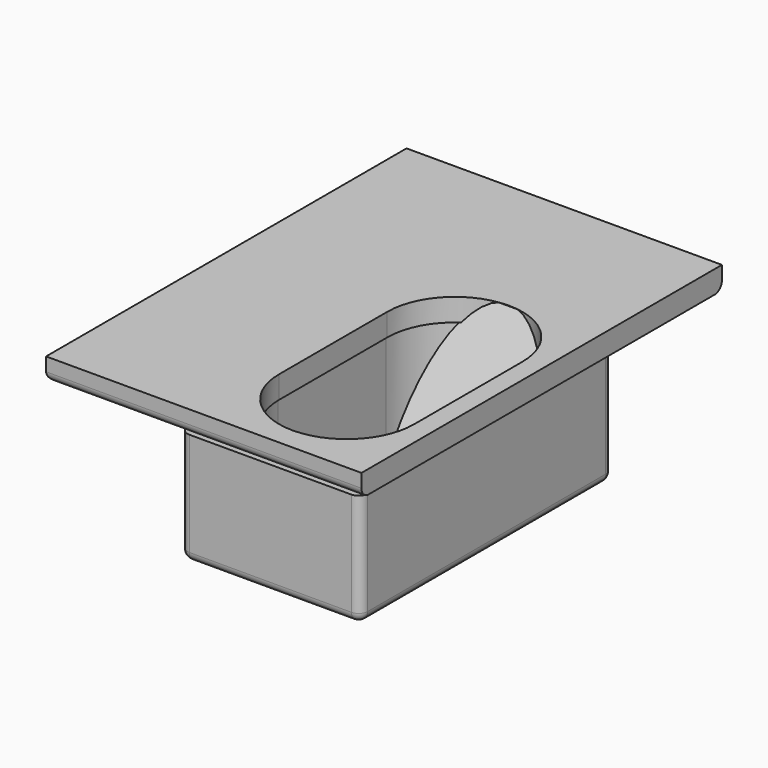
from build123d import *

# Parameters (mm, degrees)
F2_W     = 19.05
F2_H     = 25.4
F2_W_2   = 15.875
F2_H_2   = 19.05
F2_H_3   = 6.35
F2_W_3   = 6.35
F3_DEPTH = 3.175
F1_W     = 19.05
F1_H     = 6.35
F1_W_2   = 6.35
F1_H_2   = 19.05
F4_DEPTH = 15.875
F5_R     = 3.175
F6_DEPTH = 12.7
F9_DEPTH = 19.05
F10_R    = 1.27
F10_2_R  = 1.27


# Not quite as in the source:
# - a feature of the source that left no trace in its solid (it failed there, or was rolled back) is left out


with BuildPart() as f3:
    # F2 (on Top) → F3 (new body)
    with BuildSketch(Plane.XY):
        Polygon((0, 31.75), (-22.225, 31.75), (-22.225, 0), (-3.175, 0), (-3.175, 12.7), (0, 12.7), align=None)
        with Locations((-12.7, -19.05)):
            Rectangle(F2_W, F2_H)
        with Locations((14.2875, 22.225)):
            Rectangle(F2_W_2, F2_H_2)
        with Locations((-12.7, -3.175)):
            Rectangle(F2_W, F2_H_3)
        with Locations((3.175, 22.225)):
            Rectangle(F2_W_3, F2_H_2)
        Polygon((6.35, 12.7), (0, 12.7), (-3.175, 12.7), (-3.175, 0), (-3.175, -6.35), (-3.175, -31.75), (22.225, -31.75), (22.225, 12.7), align=None)
        with BuildLine():
            ThreePointArc((0.4552836776, 0), (9.9802836776, 9.525), (19.5052836776, 0))
            Line((19.5052836776, 0), (19.5052836776, -9.525))
            Line((19.5052836776, -9.525), (19.5052836776, -19.05))
            ThreePointArc((19.5052836776, -19.05), (9.9802836776, -28.575), (0.4552836776, -19.05))
            Line((0.4552836776, -19.05), (0.4552836776, -9.525))
            Line((0.4552836776, -9.525), (0.4552836776, 0))
        make_face(mode=Mode.SUBTRACT)
    extrude(amount=-F3_DEPTH)

    # F10
    f10_edges = [f3.edges().sort_by_distance(p)[0] for p in [
        (-22.225, 0, -3.175),
        (0, -31.75, -3.175),
        (0, 31.75, -3.175),
    ]]
    fillet(f10_edges, radius=F10_R)


with BuildPart() as f4:
    # F1 (on offset) → F4 (new body)
    with BuildSketch(Plane.XY.offset(-3.175)):
        with Locations((-12.8714862525, -3.1345629871)):
            Rectangle(F1_W, F1_H)
        with Locations((3.0035137475, 22.2654370129)):
            Rectangle(F1_W_2, F1_H_2)
        Polygon((6.1785137475, 12.7404370129), (-0.1714862525, 12.7404370129), (-3.3464862525, 12.7404370129), (-3.3464862525, 0.0404370129), (-3.3464862525, -6.3095629871), (-3.3464862525, -31.7095629871), (22.0535137475, -31.7095629871), (22.0535137475, 12.7404370129), align=None)
        with BuildLine():
            ThreePointArc((0.283797425, 0.0404370129), (9.808797425, 9.5654370129), (19.333797425, 0.0404370129))
            Line((19.333797425, 0.0404370129), (19.333797425, -9.4845629871))
            Line((19.333797425, -9.4845629871), (19.333797425, -19.0095629871))
            ThreePointArc((19.333797425, -19.0095629871), (9.808797425, -28.5345629871), (0.283797425, -19.0095629871))
            Line((0.283797425, -19.0095629871), (0.283797425, -9.4845629871))
            Line((0.283797425, -9.4845629871), (0.283797425, 0.0404370129))
        make_face(mode=Mode.SUBTRACT)
    extrude(amount=-F4_DEPTH)

    # F5 (on Front) → F6 (cut, symmetric)
    with BuildSketch(Plane.XZ):
        with Locations((-12.8714862525, -9.525)):
            Circle(F5_R)
    extrude(amount=F6_DEPTH, both=True, mode=Mode.SUBTRACT)

    # F10#2
    f10_2_edges = [f4.edges().sort_by_distance(p)[0] for p in [
        (-22.396486, -6.309563, -11.1125),
        (-22.396486, 0.040437, -11.1125),
        (-12.871486, 0.040437, -19.05),
        (-22.396486, -3.134563, -19.05),
        (-12.871486, -6.309563, -19.05),
        (-3.346486, -19.009563, -19.05),
        (9.353514, -31.709563, -19.05),
        (22.053514, -9.484563, -19.05),
        (14.116014, 12.740437, -19.05),
        (6.178514, 22.265437, -19.05),
        (3.003514, 31.790437, -19.05),
        (-0.171486, 22.265437, -19.05),
        (-1.758986, 12.740437, -19.05),
        (-3.346486, 6.390437, -19.05),
        (9.808797, -28.534563, -19.05),
        (0.283797, -9.484563, -19.05),
        (9.808797, 9.565437, -19.05),
        (19.333797, -9.484563, -19.05),
        (-3.346486, -31.709563, -11.1125),
        (22.053514, -31.709563, -11.1125),
        (22.053514, 12.740437, -11.1125),
        (6.178514, 31.790437, -11.1125),
    ]]
    fillet(f10_2_edges, radius=F10_2_R)


with BuildPart() as f9:
    # F7 (on Right) → F9 (new body)
    with BuildSketch(Plane.YZ):
        Polygon((9.4160083681, -19.05), (9.4160083681, 0), (0, -19.05), align=None)
    extrude(amount=F9_DEPTH)


solid = Compound([f3.part, f4.part, f9.part])
